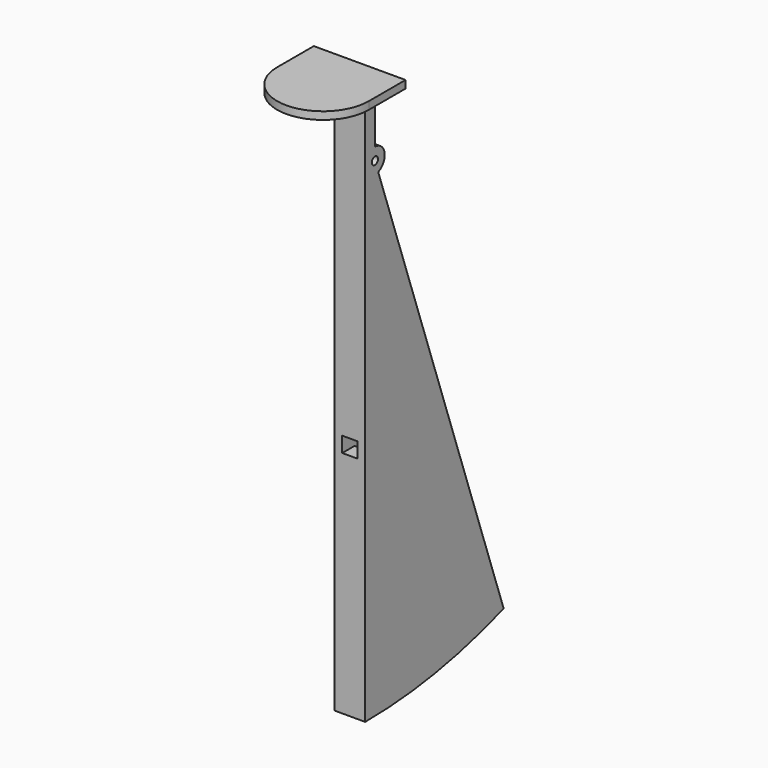
from build123d import *

# Parameters (mm, degrees)
F3_DEPTH = 1.5875
F4_R     = 0.79375
F5_DEPTH = 3.175
F6_DEPTH = 1.5875


# Not quite as in the source:
# - a length typed as a fraction of an inch, garbled in the dataset ("3 / 203.2 mm" for 3/8 in), is restored


with BuildPart() as f3:
    # F2 (on line) → F3 (new body)
    with BuildSketch(Plane(origin=(0, 0, 55.2947693627), x_dir=(1, 0, 0), z_dir=(0, 0, -1))):
        with BuildLine():
            ThreePointArc((9.525, 0), (0, 9.525), (-9.525, 0))
            Line((-9.525, 0), (-9.525, -9.525))
            Line((-9.525, -9.525), (9.525, -9.525))
            Line((9.525, -9.525), (9.525, 0))
        make_face()
    extrude(amount=-F3_DEPTH)

    # F4 (on Right) → F5 (join, symmetric)
    with BuildSketch(Plane.YZ):
        with BuildLine():
            Line((9.525, 42.5947693627), (9.525, 55.2947693627))
            Line((9.525, 55.2947693627), (6.985, 55.2947693627))
            Line((6.985, 55.2947693627), (6.985, 40.0547693627))
            ThreePointArc((6.985, 40.0547693627), (7.7289487758, 41.8508205869), (9.525, 42.5947693627))
        make_face()
        Polygon((10.16, -10.7452306373), (6.985, -10.7452306373), (6.985, -13.9202306373), (10.16, -13.9202306373), (10.16, -15.5077306373), (14.9225, -15.5077306373), (14.9225, -9.1577306373), (10.16, -9.1577306373), align=None)
        with BuildLine():
            ThreePointArc((10.3640900788, 37.6573691375), (8.0552532191, 37.9831891928), (6.985, 40.0547693627))
            Line((6.985, 40.0547693627), (6.985, -10.7452306373))
            Line((6.985, -10.7452306373), (10.16, -10.7452306373))
            Line((10.16, -10.7452306373), (10.16, -9.1577306373))
            Line((10.16, -9.1577306373), (14.9225, -9.1577306373))
            Line((14.9225, -9.1577306373), (14.9225, -15.5077306373))
            Line((14.9225, -15.5077306373), (10.16, -15.5077306373))
            Line((10.16, -15.5077306373), (10.16, -13.9202306373))
            Line((10.16, -13.9202306373), (6.985, -13.9202306373))
            Line((6.985, -13.9202306373), (6.985, -61.5452306373))
            ThreePointArc((6.985, -61.5452306373), (25.2233058777, -60.0065006912), (42.9460033775, -55.433811716))
            Line((42.9460033775, -55.433811716), (10.3640900788, 37.6573691375))
        make_face()
        with BuildLine():
            ThreePointArc((12.065, 40.0547693627), (11.3210512242, 41.8508205869), (9.525, 42.5947693627))
            ThreePointArc((9.525, 42.5947693627), (7.7289487758, 41.8508205869), (6.985, 40.0547693627))
            ThreePointArc((6.985, 40.0547693627), (8.0552532191, 37.9831891928), (10.3640900788, 37.6573691375))
            ThreePointArc((10.3640900788, 37.6573691375), (11.5965801698, 38.5850225818), (12.065, 40.0547693627))
        make_face()
        with Locations((9.525, 40.0547693627)):
            Circle(F4_R, mode=Mode.SUBTRACT)
    extrude(amount=F5_DEPTH, both=True)

    # F4 (on Right) → F6 (cut, symmetric)
    with BuildSketch(Plane.YZ):
        Polygon((10.16, -10.7452306373), (6.985, -10.7452306373), (6.985, -13.9202306373), (10.16, -13.9202306373), (10.16, -15.5077306373), (14.9225, -15.5077306373), (14.9225, -9.1577306373), (10.16, -9.1577306373), align=None)
    extrude(amount=F6_DEPTH, both=True, mode=Mode.SUBTRACT)


solid = f3.part
